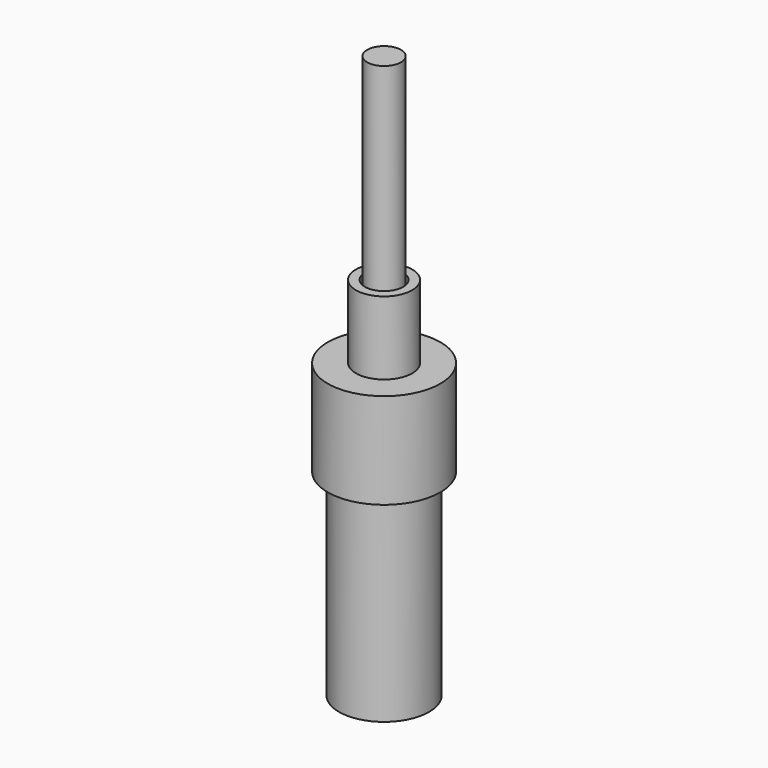
from build123d import *

# Parameters (mm, degrees)
F0_R      = 3
F1_DEPTH  = 50
F0_R_2    = 8
F2_DEPTH  = 50
F3_R      = 10
F4_DEPTH  = 15
F5_OFFSET = 0.4
F6_T      = 1.6


# Not quite as in the source:
# - a shell that OpenCascade refuses in one call is made with other operations: the cavity is built on its own and cut out


with BuildPart() as f1:
    # F0 (on Top) → F1 (new body)
    with BuildSketch(Plane.XY):
        Circle(F0_R)
    extrude(amount=F1_DEPTH)

    # F0 (on Top) → F2 (join)
    with BuildSketch(Plane.XY):
        Circle(F0_R_2)
        Circle(F0_R, mode=Mode.SUBTRACT)
        Circle(F0_R)
    extrude(amount=-F2_DEPTH)


with BuildPart() as f4:
    # F3 (on face) → F4 (new body, symmetric)
    with BuildSketch(Plane.XY):
        Circle(F3_R)
    extrude(amount=F4_DEPTH, both=True)

    # F5: cut F1, made larger all round first
    f5_tool = offset(f1.part, amount=F5_OFFSET, kind=Kind.INTERSECTION, mode=Mode.PRIVATE)
    add(f5_tool, mode=Mode.SUBTRACT)

    # F6: shell of thickness 1.6, made by hand


with BuildPart() as f6_core1:
    # F6_t2: copy of F4
    add(f4.part)

    # the walls: a layer under each face that stays
    f6_faces = [f6_core1.faces().sort_by_distance(p)[0] for p in [
        (-6.6666666667, -6.6666666667, -15),
        (-8.4, 0, -7.3),
        (-3.4, 0, 7.7),
        (-5.6, -5.6, 0.4),
    ]]
    thicken(f6_faces, amount=-F6_T, mode=Mode.SUBTRACT)

    # F6_s3 → F6_t4 (revolve, cut)
    with BuildSketch(Plane.XZ):
        Polygon((8.384, 0.384), (10, 0.4), (10, 2), (8.4, 2), align=None)
    revolve(axis=Axis((0, 0, 0.4), (0, 0, 1)), mode=Mode.SUBTRACT)


with BuildPart() as f4_1:
    add(f4.part)

    # what is left inside the walls is the cavity
    f6_cavity = [f6_core1.part.solids().sort_by_distance(p)[0] for p in [
        (-9.984, 0, 6.333333),
    ]]
    add(f6_cavity, mode=Mode.SUBTRACT)


solid = Compound([f1.part, f4_1.part])
